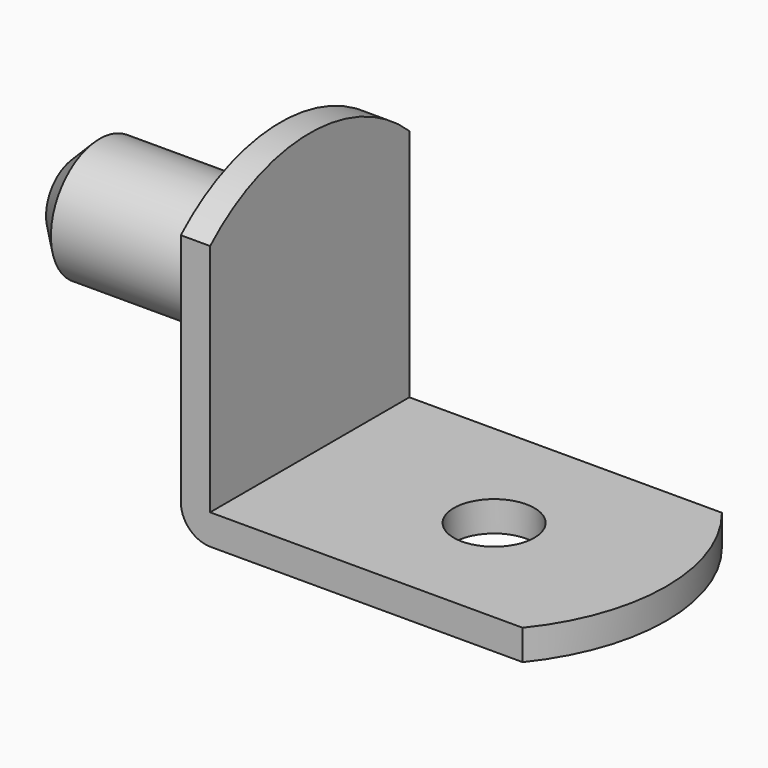
from build123d import *

# Parameters (mm, degrees)
F0_W     = 12.954
F0_H     = 12.192
F0_R     = 3.175
F0_H_2   = 1.5748
F1_DEPTH = 1.524
F2_DEPTH = 12.192
F3_SIZE  = 1.27
F5_W     = 16.256
F5_H     = 12.954
F5_R     = 2.0955
F6_DEPTH = 1.5748
F7_R     = 1.5494


# Not quite as in the source:
# - a feature names something its author has since deleted; it is built from what else it names


with BuildPart() as f1:
    # F0 (on Right) → F1 (new body)
    with BuildSketch(Plane.YZ):
        with BuildLine():
            ThreePointArc((6.477, 6.096), (0, 8.636), (-6.477, 6.096))
            Line((-6.477, 6.096), (6.477, 6.096))
        make_face()
        Rectangle(F0_W, F0_H)
        with Locations((0, 1.651)):
            Circle(F0_R, mode=Mode.SUBTRACT)
        with Locations((0, -6.8834)):
            Rectangle(F0_W, F0_H_2)
        with Locations((0, 1.651)):
            Circle(F0_R)
    extrude(amount=-F1_DEPTH)

    # F0 (on Right) → F2 (join)
    with BuildSketch(Plane.YZ):
        with Locations((0, 1.651)):
            Circle(F0_R)
    extrude(amount=-F2_DEPTH)

    # F3
    f3_edges = [f1.edges().sort_by_distance(p)[0] for p in [
        (-12.192, -3.175, 1.651),
    ]]
    chamfer(f3_edges, length=F3_SIZE)

    # F5 (on offset) → F6 (join)
    with BuildSketch(Plane(origin=(0, 0, -7.6708), x_dir=(1, 0, 0), z_dir=(0, 0, -1))):
        with Locations((8.128, 0)):
            Rectangle(F5_W, F5_H)
        with Locations((9.5885, 0)):
            Circle(F5_R, mode=Mode.SUBTRACT)
        with BuildLine():
            Line((16.256, 6.477), (16.256, -6.477))
            ThreePointArc((16.256, -6.477), (18.542, 0), (16.256, 6.477))
        make_face()
    extrude(amount=-F6_DEPTH)

    # F7
    f7_edges = [f1.edges().sort_by_distance(p)[0] for p in [
        (-1.524, 0, -7.6708),
    ]]
    fillet(f7_edges, radius=F7_R)


solid = f1.part
